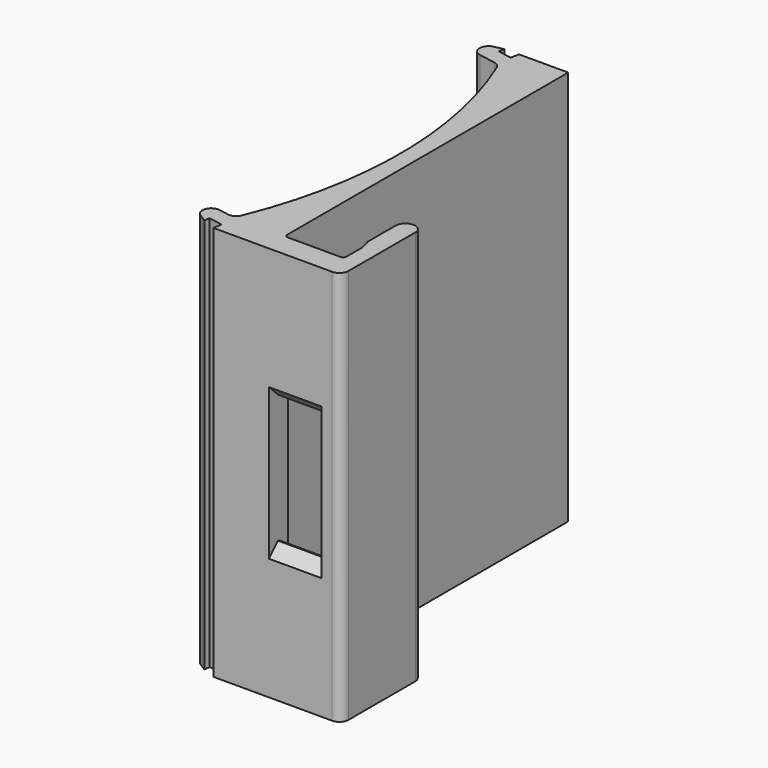
from build123d import *

# Parameters (mm, degrees)
F0_W     = 9
F0_H     = 2.6991704602
F0_H_2   = 1.5
F1_DEPTH = 70
F2_R     = 1.55
F3_W     = 9.3
F3_H     = 22.7586206897
F4_DEPTH = 5
F5_SIZE  = 2
F6_R     = 0.59999
F7_R     = 1.6


# Not quite as in the source:
# - a fillet or chamfer is up to 0.001 mm smaller than in the source, because OpenCascade refuses the exact size
# - a feature names something its author has since deleted; it is built from what else it names


with BuildPart() as f1:
    # F0 (on Top) → F1 (new body)
    with BuildSketch(Plane.XY):
        Polygon((-9, -32), (-9, -29.3008295398), (-13.4364079285, -28.4836487781), (-13.9172762663, -31.0942438952), (-11.4586381331, -31.5471219476), align=None)
        with Locations((-4.5, -30.6504147699)):
            Rectangle(F0_W, F0_H)
        Polygon((-9, -33.5), (-9, -32), (-9.2639088239, -33.5), align=None)
        with Locations((-4.5, -32.75)):
            Rectangle(F0_W, F0_H_2)
        Polygon((-11.6319159151, -32.5319949396), (-11.4586381331, -31.5471219476), (-13.9172762663, -31.0942438952), align=None)
        with BuildLine():
            Line((0, -29.3008295398), (0, 29.3008295398))
            Line((0, 29.3008295398), (-9, 29.3008295398))
            ThreePointArc((-9, 29.3008295398), (-2.9680403173, 0), (-9, -29.3008295398))
            Line((-9, -29.3008295398), (0, -29.3008295398))
        make_face()
        with Locations((-4.5, 30.6504147699)):
            Rectangle(F0_W, F0_H)
        Polygon((0, 32), (0, 33.5), (-8.7112760279, 33.5), (-9, 32), align=None)
        Polygon((-9, 29.3008295398), (-9, 32), (-11.4586381331, 32.4528780524), (-13.9172762663, 32.9057561048), (-14.398144604, 30.2951609877), align=None)
        Polygon((-13.9172762663, 32.9057561048), (-11.4586381331, 32.4528780524), (-11.2696250671, 33.4348526248), align=None)
        Polygon((10.5, -29.3008295398), (0, -29.3008295398), (0, -32), (0, -33.5), (13.4, -33.5), (13.4, -15.5), (10.7962751514, -15.5), (10.5, -15.9545544746), (10.5, -22.238118574), (10.5, -25.2114422619), align=None)
        Polygon((10, -23.3806278557), (10.5, -25.2114422619), (10.5, -22.238118574), (10.5, -15.9545544746), (10, -16.7216698947), align=None)
    extrude(amount=F1_DEPTH)

    # F2
    f2_edges = [f1.edges().sort_by_distance(p)[0] for p in [
        (-14.398145, 30.295161, 35),
        (-9, 29.30083, 35),
        (-13.436408, -28.483649, 35),
        (-9, -29.30083, 35),
        (-13.917276, -31.094244, 35),
        (-13.917276, 32.905756, 35),
    ]]
    fillet(f2_edges, radius=F2_R)

    # F3 (on face) → F4 (cut)
    with BuildSketch(Plane.XZ.offset(33.5)):
        with Locations((5.25, 35)):
            Rectangle(F3_W, F3_H)
    extrude(amount=-F4_DEPTH, mode=Mode.SUBTRACT)

    # F5
    f5_edges = [f1.edges().sort_by_distance(p)[0] for p in [
        (5.25, -33.5, 46.37931),
        (5.25, -33.5, 23.62069),
        (5.25, -29.30083, 23.62069),
        (5.25, -29.30083, 46.37931),
    ]]
    chamfer(f5_edges, length=F5_SIZE)

    # F6 (radius 0.6 in the source; OpenCascade refuses exactly that, so slightly less here)
    f6_edges = [f1.edges().sort_by_distance(p)[0] for p in [
        (0, -29.30083, 35),
        (10.5, -29.30083, 35),
    ]]
    fillet(f6_edges, radius=F6_R)

    # F7
    f7_edges = [f1.edges().sort_by_distance(p)[0] for p in [
        (10.796275, -15.5, 35),
        (13.4, -15.5, 35),
        (10, -16.72167, 35),
        (13.4, -33.5, 35),
    ]]
    fillet(f7_edges, radius=F7_R)


solid = f1.part
